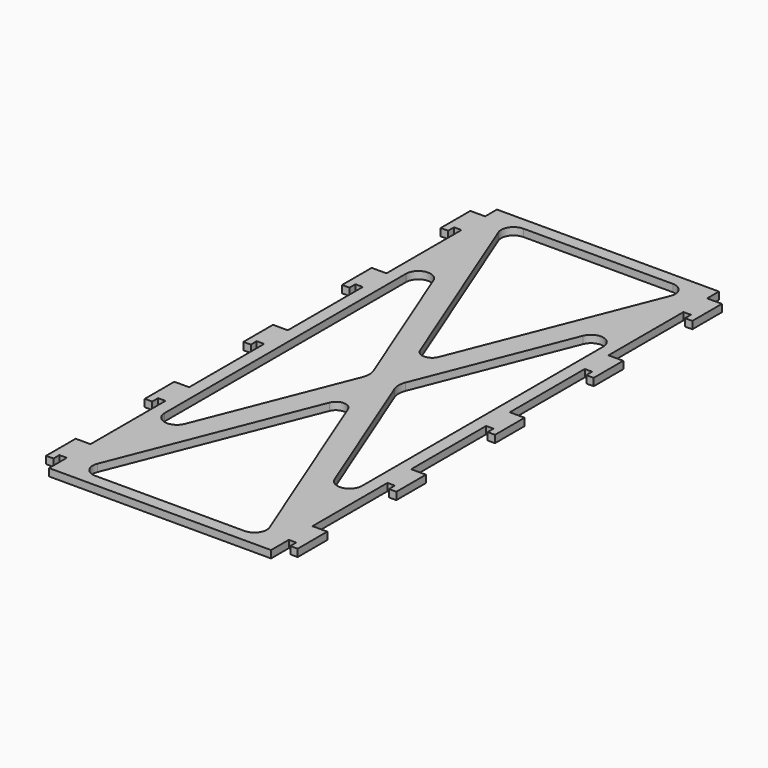
from build123d import *

# Parameters (mm, degrees)
F0_W     = 90
F0_H     = 227
F1_DEPTH = 3
F3_DEPTH = 3


# Not quite as in the source:
# - a feature names something its author has since deleted; it is built from what else it names


with BuildPart() as f1:
    # F0 (on Top) → F1 (new body)
    with BuildSketch(Plane.XY):
        Rectangle(F0_W, F0_H)
        with BuildLine():
            ThreePointArc((-30.2779513906, -108.4999991059), (-34.4140194322, -106.3094369778), (-34.9259618692, -101.6571755682))
            Line((-34.9259618692, -101.6571755682), (-3.7184084714, -22.9447908871))
            ThreePointArc((-3.7184084714, -22.9447908871), (-8.85e-08, -20.4190497173), (3.7184082943, -22.9447908871))
            Line((3.7184082943, -22.9447908871), (34.9259616921, -101.6571755682))
            ThreePointArc((34.9259616921, -101.6571755682), (34.4140192551, -106.3094369778), (30.2779512136, -108.4999991059))
            Line((30.2779512136, -108.4999991059), (-30.2779513906, -108.4999991059))
        make_face(mode=Mode.SUBTRACT)
        with BuildLine():
            ThreePointArc((-40, 61.145500066), (-35.9380691891, 66.0567143962), (-30.3519895215, 62.9883236038))
            Line((-30.3519895215, 62.9883236038), (-6.4745976856, 2.7642353066))
            ThreePointArc((-6.4745976856, 2.7642353066), (-5.9466134034, 0), (-6.4745976856, -2.7642353066))
            Line((-6.4745976856, -2.7642353066), (-30.3519895215, -62.9883236038))
            ThreePointArc((-30.3519895214, -62.9883236038), (-35.9380691891, -66.0567143962), (-40, -61.145500066))
            Line((-40, -61.145500066), (-40, 61.145500066))
        make_face(mode=Mode.SUBTRACT)
        with BuildLine():
            ThreePointArc((30.2779512136, 108.4999991059), (34.4140192551, 106.3094369778), (34.9259616921, 101.6571755682))
            Line((34.9259616921, 101.6571755682), (3.7184082943, 22.9447908871))
            ThreePointArc((3.7184082943, 22.9447908871), (-8.85e-08, 20.4190497173), (-3.7184084714, 22.9447908871))
            Line((-3.7184084714, 22.9447908871), (-34.9259618692, 101.6571755682))
            ThreePointArc((-34.9259618692, 101.6571755682), (-34.4140194322, 106.3094369778), (-30.2779513906, 108.4999991059))
            Line((-30.2779513906, 108.4999991059), (30.2779512136, 108.4999991059))
        make_face(mode=Mode.SUBTRACT)
        with BuildLine():
            Line((6.4745976856, 2.7642353066), (30.3519895215, 62.9883236038))
            ThreePointArc((30.3519895215, 62.9883236038), (35.9380691891, 66.0567143962), (40, 61.145500066))
            Line((40, 61.145500066), (40, -61.145500066))
            ThreePointArc((40, -61.145500066), (35.9380691891, -66.0567143962), (30.3519895214, -62.9883236038))
            Line((30.3519895215, -62.9883236038), (6.4745976856, -2.7642353066))
            ThreePointArc((6.4745976856, -2.7642353066), (5.9466134034, 0), (6.4745976856, 2.7642353066))
        make_face(mode=Mode.SUBTRACT)
    extrude(amount=F1_DEPTH)

    # F2 (on face) → F3 (join, through all)
    with BuildSketch(Plane.XY.offset(3)):
        Polygon((-45, 95.5), (-45, 107.5), (-51, 107.5), (-51, 92.5), (-48, 92.5), (-48, 95.5), align=None)
        Polygon((51, 107.5), (45, 107.5), (45, 95.5), (48, 95.5), (48, 92.5), (51, 92.5), align=None)
        Polygon((-45, 45.5), (-45, 57.5), (-51, 57.5), (-51, 42.5), (-48, 42.5), (-48, 45.5), align=None)
        Polygon((51, 57.5), (45, 57.5), (45, 45.5), (48, 45.5), (48, 42.5), (51, 42.5), align=None)
        Polygon((-45, 113.5), (-45, 107.5), (-45, 95.5), (-45, 57.5), (-45, 45.5), (-45, 7.5), (-45, -4.5), (-45, -42.5), (-45, -54.5), (-45, -92.5), (-45, -104.5), (-45, -113.5), (45, -113.5), (45, -104.5), (45, -92.5), (45, -54.5), (45, -42.5), (45, -4.5), (45, 7.5), (45, 45.5), (45, 57.5), (45, 95.5), (45, 107.5), (45, 113.5), align=None)
        with BuildLine():
            Line((3.7184082943, -22.9447908871), (34.9259616921, -101.6571755682))
            ThreePointArc((34.9259616921, -101.6571755682), (34.4140192551, -106.3094369778), (30.2779512136, -108.4999991059))
            Line((30.2779512136, -108.4999991059), (-30.2779513906, -108.4999991059))
            ThreePointArc((-30.2779513906, -108.4999991059), (-34.4140194322, -106.3094369778), (-34.9259618692, -101.6571755682))
            Line((-34.9259618692, -101.6571755682), (-3.7184084714, -22.9447908871))
            ThreePointArc((-3.7184084714, -22.9447908871), (-8.85e-08, -20.4190497173), (3.7184082943, -22.9447908871))
        make_face(mode=Mode.SUBTRACT)
        with BuildLine():
            ThreePointArc((-30.3519895214, -62.9883236038), (-35.9380691891, -66.0567143962), (-40, -61.145500066))
            Line((-40, -61.145500066), (-40, 61.145500066))
            ThreePointArc((-40, 61.145500066), (-35.9380691891, 66.0567143962), (-30.3519895215, 62.9883236038))
            Line((-30.3519895215, 62.9883236038), (-6.4745976856, 2.7642353066))
            ThreePointArc((-6.4745976856, 2.7642353066), (-5.9466134034, 0), (-6.4745976856, -2.7642353066))
            Line((-6.4745976856, -2.7642353066), (-30.3519895215, -62.9883236038))
        make_face(mode=Mode.SUBTRACT)
        with BuildLine():
            ThreePointArc((-34.9259618692, 101.6571755682), (-34.4140194322, 106.3094369778), (-30.2779513906, 108.4999991059))
            Line((-30.2779513906, 108.4999991059), (30.2779512136, 108.4999991059))
            ThreePointArc((30.2779512136, 108.4999991059), (34.4140192551, 106.3094369778), (34.9259616921, 101.6571755682))
            Line((34.9259616921, 101.6571755682), (3.7184082943, 22.9447908871))
            ThreePointArc((3.7184082943, 22.9447908871), (-8.85e-08, 20.4190497173), (-3.7184084714, 22.9447908871))
            Line((-3.7184084714, 22.9447908871), (-34.9259618692, 101.6571755682))
        make_face(mode=Mode.SUBTRACT)
        with BuildLine():
            ThreePointArc((6.4745976856, -2.7642353066), (5.9466134034, 0), (6.4745976856, 2.7642353066))
            Line((6.4745976856, 2.7642353066), (30.3519895215, 62.9883236038))
            ThreePointArc((30.3519895215, 62.9883236038), (35.9380691891, 66.0567143962), (40, 61.145500066))
            Line((40, 61.145500066), (40, -61.145500066))
            ThreePointArc((40, -61.145500066), (35.9380691891, -66.0567143962), (30.3519895214, -62.9883236038))
            Line((30.3519895215, -62.9883236038), (6.4745976856, -2.7642353066))
        make_face(mode=Mode.SUBTRACT)
        Polygon((-45, -4.5), (-45, 7.5), (-51, 7.5), (-51, -7.5), (-48, -7.5), (-48, -4.5), align=None)
        Polygon((-45, -54.5), (-45, -42.5), (-51, -42.5), (-51, -57.5), (-48, -57.5), (-48, -54.5), align=None)
        Polygon((-45, -104.5), (-45, -92.5), (-51, -92.5), (-51, -107.5), (-48, -107.5), (-48, -104.5), align=None)
        Polygon((51, -92.5), (45, -92.5), (45, -104.5), (48, -104.5), (48, -107.5), (51, -107.5), align=None)
        Polygon((51, -42.5), (45, -42.5), (45, -54.5), (48, -54.5), (48, -57.5), (51, -57.5), align=None)
        Polygon((51, 7.5), (45, 7.5), (45, -4.5), (48, -4.5), (48, -7.5), (51, -7.5), align=None)
    extrude(amount=-F3_DEPTH)


solid = f1.part
